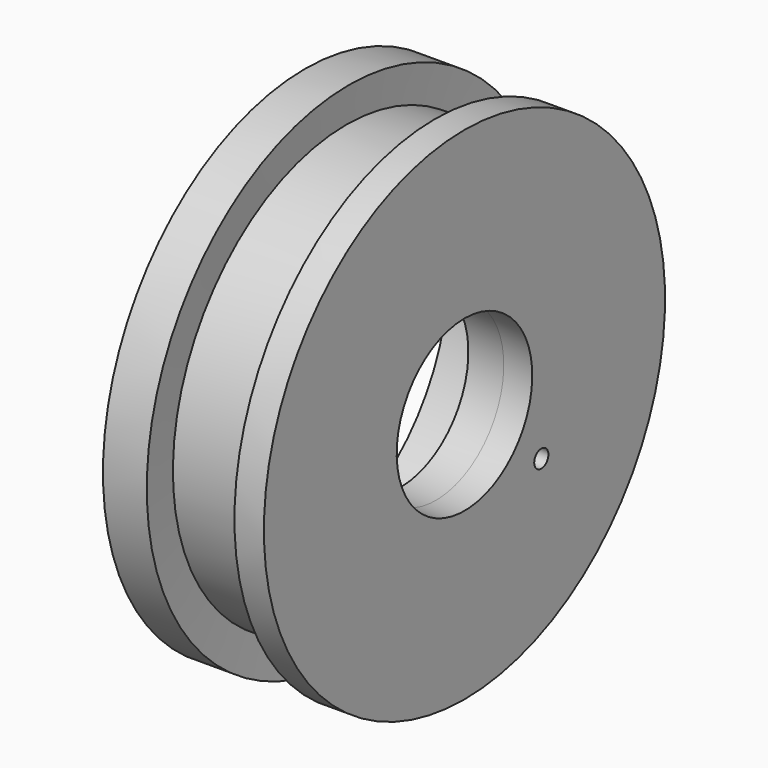
from build123d import *
from build123d import SkipClean  # not in build123d's __all__

# Parameters (mm, degrees)
F4_D     = 12.7
F5_R     = 128.2794587314
F5_R_2   = 6.35
F5_R_3   = 60.7691295445
F6_DEPTH = 25.4


with BuildPart() as f2:
    # F0 (on Front) → F2 (revolve)
    with BuildSketch(Plane.XZ):
        Polygon((-52.4943843484, 27.3255631328), (-32.0674665272, 27.3255631328), (-32.0674665272, 113.4814321995), (-32.0674665272, 146.3606357574), (-53.1988926232, 146.3606357574), (-53.1988926232, 122.2296878695), (-116.6306659579, 122.2296878695), (-114.9781197309, 147.7223485708), (-146.413102746, 147.7223485708), (-146.413102746, 94.8358923197), (-52.4943843484, 94.8358923197), align=None)
    revolve(axis=Axis((-79.9387739971, 0, -33.4435664117), (1, 0, 0)))

    # F4 (through all)
    with Locations(Plane(origin=(-52.4943843484, 0, 0), x_dir=(0, -1, 0), z_dir=(-1, 0, 0))):
        with Locations((-68.8715130091, -89.2082676291)):
            Hole(F4_D / 2)

    # F5 (on face) → F6 (join)
    with BuildSketch(Plane(origin=(-52.4943843484, 0, 0), x_dir=(0, -1, 0), z_dir=(-1, 0, 0))):
        with Locations((0, -33.4435664117)):
            Circle(F5_R)
        with Locations((-68.8715130091, -89.2082676291)):
            Circle(F5_R_2, mode=Mode.SUBTRACT)
        with Locations((0, -33.4435664117)):
            Circle(F5_R_3, mode=Mode.SUBTRACT)
    with SkipClean():  # cleaning this boolean's faces spoils the solid; the shape is the same uncleaned
        extrude(amount=F6_DEPTH)


solid = f2.part
